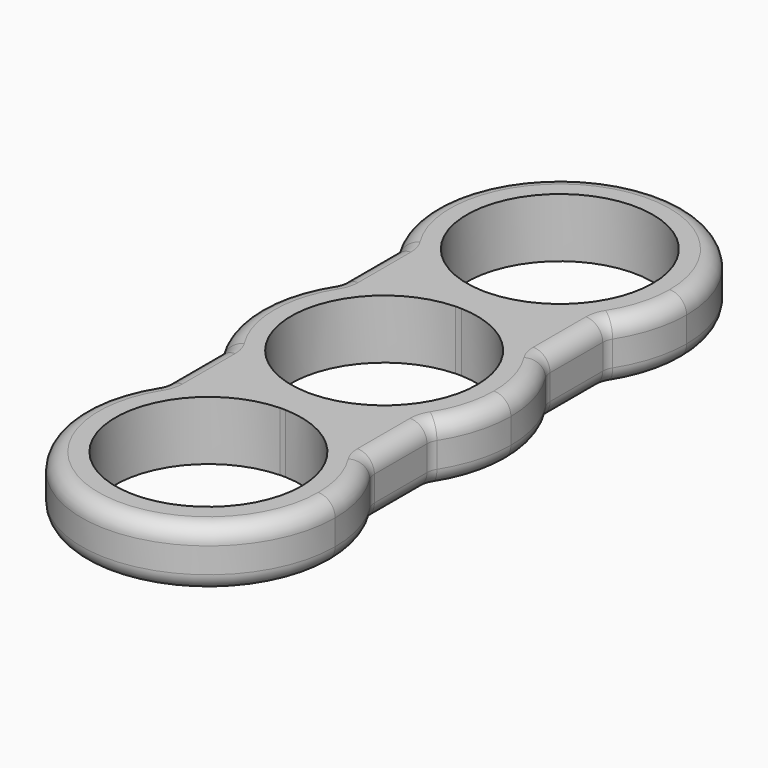
from build123d import *

# Parameters (mm, degrees)
F1_DEPTH = 7
F2_F1_R  = 2
F2_F2_R  = 2


with BuildPart() as f1:
    # F0 (on Top) → F1 (new body)
    with BuildSketch(Plane.XY):
        with BuildLine():
            ThreePointArc((0.3357339129, 14.9962422873), (4.0392104898, 14.4459260215), (7.4910247439, 12.9955587909))
            ThreePointArc((7.4910247439, 12.9955587909), (10.1759290258, 14.9706607644), (12.3583803583, 17.4899156126))
            ThreePointArc((12.3583803583, 17.4899156126), (14.3243796615, 21.540033746), (15, 25.9911175817))
            ThreePointArc((15, 25.9911175817), (-4.4510838357, 40.3154972432), (-12.3583803583, 17.4899156126))
            ThreePointArc((-12.3583803583, 17.4899156126), (-10.1759290258, 14.9706607644), (-7.4910247439, 12.9955587909))
            ThreePointArc((-7.4910247439, 12.9955587909), (-4.0392104898, 14.4459260215), (-0.3357339129, 14.9962422873))
            ThreePointArc((-0.3357339129, 14.9962422873), (-7.6585549211, 33.8870998842), (11, 25.9911175817))
            ThreePointArc((11, 25.9911175817), (7.8959823025, 18.3325626607), (0.3357339129, 14.9962422873))
        make_face()
        with BuildLine():
            ThreePointArc((-0.3357339129, 10.9948752944), (0, 11), (0.3357339129, 10.9948752944))
            ThreePointArc((0.3357339129, 10.9948752944), (4.0392104898, 11.5451915602), (7.4910247439, 12.9955587909))
            ThreePointArc((7.4910247439, 12.9955587909), (4.0392104898, 14.4459260215), (0.3357339129, 14.9962422873))
            ThreePointArc((0.3357339129, 14.9962422873), (0, 14.9911175817), (-0.3357339129, 14.9962422873))
            ThreePointArc((-0.3357339129, 14.9962422873), (-4.0392104898, 14.4459260215), (-7.4910247439, 12.9955587909))
            ThreePointArc((-7.4910247439, 12.9955587909), (-4.0392104898, 11.5451915602), (-0.3357339129, 10.9948752944))
        make_face()
        with BuildLine():
            ThreePointArc((12.3583803583, 17.4899156126), (10.1759290258, 14.9706607644), (7.4910247439, 12.9955587909))
            ThreePointArc((7.4910247439, 12.9955587909), (10.1759290258, 11.0204568173), (12.3583803583, 8.5012019691))
            Line((12.3583803583, 8.5012019691), (12.3583803583, 17.4899156126))
        make_face()
        with BuildLine():
            ThreePointArc((-12.3583803583, 8.5012019691), (-10.1759290258, 11.0204568173), (-7.4910247439, 12.9955587909))
            ThreePointArc((-7.4910247439, 12.9955587909), (-10.1759290258, 14.9706607644), (-12.3583803583, 17.4899156126))
            Line((-12.3583803583, 17.4899156126), (-12.3583803583, 8.5012019691))
        make_face()
        with BuildLine():
            ThreePointArc((-0.3357339129, -10.9948752944), (-11, 0), (-0.3357339129, 10.9948752944))
            ThreePointArc((-0.3357339129, 10.9948752944), (-4.0392104898, 11.5451915602), (-7.4910247439, 12.9955587909))
            ThreePointArc((-7.4910247439, 12.9955587909), (-10.1759290258, 11.0204568173), (-12.3583803583, 8.5012019691))
            ThreePointArc((-12.3583803583, 8.5012019691), (-15, 0), (-12.3583803583, -8.5012019691))
            ThreePointArc((-12.3583803583, -8.5012019691), (-10.1759290258, -11.0204568173), (-7.4910247439, -12.9955587909))
            ThreePointArc((-7.4910247439, -12.9955587909), (-4.0392104898, -11.5451915602), (-0.3357339129, -10.9948752944))
        make_face()
        with BuildLine():
            ThreePointArc((12.3583803583, -8.5012019691), (10.1759290258, -11.0204568173), (7.4910247439, -12.9955587909))
            ThreePointArc((7.4910247439, -12.9955587909), (10.1759290258, -14.9706607644), (12.3583803583, -17.4899156126))
            Line((12.3583803583, -17.4899156126), (12.3583803583, -8.5012019691))
        make_face()
        with BuildLine():
            ThreePointArc((-12.3583803583, -17.4899156126), (-10.1759290258, -14.9706607644), (-7.4910247439, -12.9955587909))
            ThreePointArc((-7.4910247439, -12.9955587909), (-10.1759290258, -11.0204568173), (-12.3583803583, -8.5012019691))
            Line((-12.3583803583, -8.5012019691), (-12.3583803583, -17.4899156126))
        make_face()
        with BuildLine():
            ThreePointArc((7.4910247439, -12.9955587909), (4.0392104898, -11.5451915602), (0.3357339129, -10.9948752944))
            ThreePointArc((0.3357339129, -10.9948752944), (0, -11), (-0.3357339129, -10.9948752944))
            ThreePointArc((-0.3357339129, -10.9948752944), (-4.0392104898, -11.5451915602), (-7.4910247439, -12.9955587909))
            ThreePointArc((-7.4910247439, -12.9955587909), (-4.0392104898, -14.4459260215), (-0.3357339129, -14.9962422873))
            ThreePointArc((-0.3357339129, -14.9962422873), (0, -14.9911175817), (0.3357339129, -14.9962422873))
            ThreePointArc((0.3357339129, -14.9962422873), (4.0392104898, -14.4459260215), (7.4910247439, -12.9955587909))
        make_face()
        with BuildLine():
            ThreePointArc((12.3583803583, -17.4899156126), (10.1759290258, -14.9706607644), (7.4910247439, -12.9955587909))
            ThreePointArc((7.4910247439, -12.9955587909), (4.0392104898, -14.4459260215), (0.3357339129, -14.9962422873))
            ThreePointArc((0.3357339129, -14.9962422873), (7.8959823025, -18.3325626607), (11, -25.9911175817))
            ThreePointArc((11, -25.9911175817), (-7.6585549211, -33.8870998842), (-0.3357339129, -14.9962422873))
            ThreePointArc((-0.3357339129, -14.9962422873), (-4.0392104898, -14.4459260215), (-7.4910247439, -12.9955587909))
            ThreePointArc((-7.4910247439, -12.9955587909), (-10.1759290258, -14.9706607644), (-12.3583803583, -17.4899156126))
            ThreePointArc((-12.3583803583, -17.4899156126), (-4.4510838357, -40.3154972432), (15, -25.9911175817))
            ThreePointArc((15, -25.9911175817), (14.3243796615, -21.540033746), (12.3583803583, -17.4899156126))
        make_face()
        with BuildLine():
            ThreePointArc((0.3357339129, 10.9948752944), (7.8959823025, 7.6585549211), (11, 0))
            ThreePointArc((11, 0), (7.8959823025, -7.6585549211), (0.3357339129, -10.9948752944))
            ThreePointArc((0.3357339129, -10.9948752944), (4.0392104898, -11.5451915602), (7.4910247439, -12.9955587909))
            ThreePointArc((7.4910247439, -12.9955587909), (10.1759290258, -11.0204568173), (12.3583803583, -8.5012019691))
            ThreePointArc((12.3583803583, -8.5012019691), (14.3243796615, -4.4510838357), (15, 0))
            ThreePointArc((15, 0), (14.3243796615, 4.4510838357), (12.3583803583, 8.5012019691))
            ThreePointArc((12.3583803583, 8.5012019691), (10.1759290258, 11.0204568173), (7.4910247439, 12.9955587909))
            ThreePointArc((7.4910247439, 12.9955587909), (4.0392104898, 11.5451915602), (0.3357339129, 10.9948752944))
        make_face()
    extrude(amount=F1_DEPTH)

    # F2: fillet of radius 2 on 16 edges, made by hand

    # F2_f1
    f2_f1_edges = [f1.edges().sort_by_distance(p)[0] for p in [
        (-12.3583803583, -17.4899156126, 3.5),
        (12.3583803583, -17.4899156126, 3.5),
        (12.3583803583, -8.5012019691, 3.5),
        (12.3583803583, 8.5012019691, 3.5),
        (12.3583803583, 17.4899156126, 3.5),
        (-12.3583803583, 17.4899156126, 3.5),
        (-12.3583803583, 8.5012019691, 3.5),
        (-12.3583803583, -8.5012019691, 3.5),
    ]]
    fillet(f2_f1_edges, radius=F2_F1_R)

    # F2_f2
    f2_f2_edges = [f1.edges().sort_by_distance(p)[0] for p in [
        (0, -40.9911175817, 0),
        (0, -40.9911175817, 7),
        (15, 0, 0),
        (15, 0, 7),
        (0, 40.9911175817, 0),
        (0, 40.9911175817, 7),
        (-15, 0, 0),
        (-15, 0, 7),
        (-12.4376458065, 8.5440032789, 7),
        (-12.4376458065, -8.5440032789, 7),
        (-12.4376458065, 8.5440032789, 0),
        (-12.4376458065, -8.5440032789, 0),
        (12.4376458065, 17.4471143028, 7),
        (-12.4376458065, 17.4471143028, 7),
        (12.4376458065, 17.4471143028, 0),
        (-12.4376458065, 17.4471143028, 0),
        (12.4376458065, -8.5440032789, 7),
        (12.4376458065, 8.5440032789, 7),
        (12.4376458065, -8.5440032789, 0),
        (12.4376458065, 8.5440032789, 0),
        (-12.4376458065, -17.4471143028, 7),
        (12.4376458065, -17.4471143028, 7),
        (-12.4376458065, -17.4471143028, 0),
        (12.4376458065, -17.4471143028, 0),
    ]]
    fillet(f2_f2_edges, radius=F2_F2_R)


solid = f1.part
